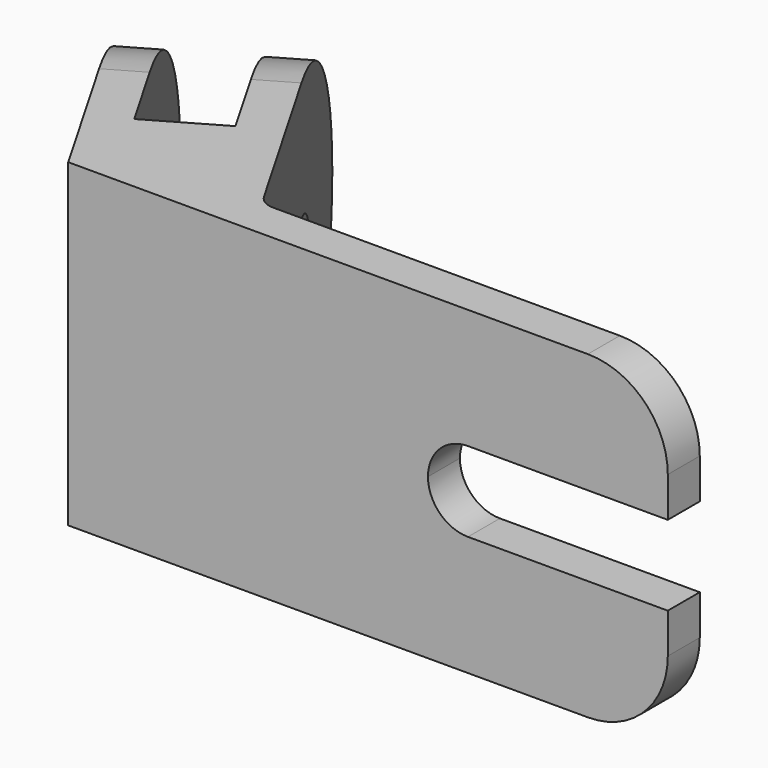
from build123d import *

# Parameters (mm, degrees)
F1_DEPTH = 80
F3_DEPTH = 36
F4_R     = 20
F5_R     = 5
F6_R     = 39.99999
F8_DEPTH = 85


# Not quite as in the source:
# - a fillet or chamfer is up to 0.001 mm smaller than in the source, because OpenCascade refuses the exact size


with BuildPart() as f1:
    # F0 (on Top) → F1 (new body)
    with BuildSketch(Plane.XY):
        Polygon((-40, 69.2820323028), (0, 0), (150, 0), (150, 10), (40.4145188433, 10), (-5.3589838486, 89.2820323028), (-14.0192378865, 84.2820323028), (15.9807621135, 32.3205080757), (-1.3397459622, 22.3205080757), (-31.3397459622, 74.2820323028), align=None)
    extrude(amount=F1_DEPTH)

    # F2 (on face) → F3 (cut)
    with BuildSketch(Plane(origin=(0, 10, 0), x_dir=(-1, 0, 0), z_dir=(0, 1, 0))):
        with BuildLine():
            Line((-90, 40), (-150, 40))
            Line((-150, 40), (-150, 30))
            Line((-150, 30), (-100, 30))
            ThreePointArc((-100, 30), (-92.9289321881, 32.9289321881), (-90, 40))
        make_face()
        with BuildLine():
            Line((-150, 50), (-150, 40))
            Line((-150, 40), (-90, 40))
            ThreePointArc((-90, 40), (-92.9289321881, 47.0710678119), (-100, 50))
            Line((-100, 50), (-150, 50))
        make_face()
    extrude(amount=-F3_DEPTH, mode=Mode.SUBTRACT)

    # F4
    f4_edges = [f1.edges().sort_by_distance(p)[0] for p in [
        (150, 5, 80),
        (150, 5, 0),
    ]]
    fillet(f4_edges, radius=F4_R)

    # F5
    f5_edges = [f1.edges().sort_by_distance(p)[0] for p in [
        (40.414519, 10, 40),
    ]]
    fillet(f5_edges, radius=F5_R)

    # F6 (radius 40 in the source; OpenCascade refuses exactly that, so slightly less here)
    f6_edges = [f1.edges().sort_by_distance(p)[0] for p in [
        (-9.689111, 86.782032, 0),
        (-35.669873, 71.782032, 0),
        (-9.689111, 86.782032, 80),
        (-35.669873, 71.782032, 80),
    ]]
    fillet(f6_edges, radius=F6_R)

    # F7 (on face) → F8 (cut)
    with BuildSketch(Plane(origin=(34.6410161514, 20, 0), x_dir=(-0.5, 0.8660254038, 0), z_dir=(0.8660254038, 0.5, 0))):
        with BuildLine():
            ThreePointArc((50.0682017207, 40), (47.1151153286, 47.0951397875), (40, 49.9997674236))
            ThreePointArc((40, 49.9997674236), (32.9730619333, 47.0469136078), (30.0682017207, 40))
            ThreePointArc((30.0682017207, 40), (32.9730619333, 32.9530863922), (40, 30.0002325764))
            ThreePointArc((40, 30.0002325764), (47.1151153286, 32.9048602125), (50.0682017207, 40))
        make_face()
    extrude(amount=-F8_DEPTH, mode=Mode.SUBTRACT)


solid = f1.part
